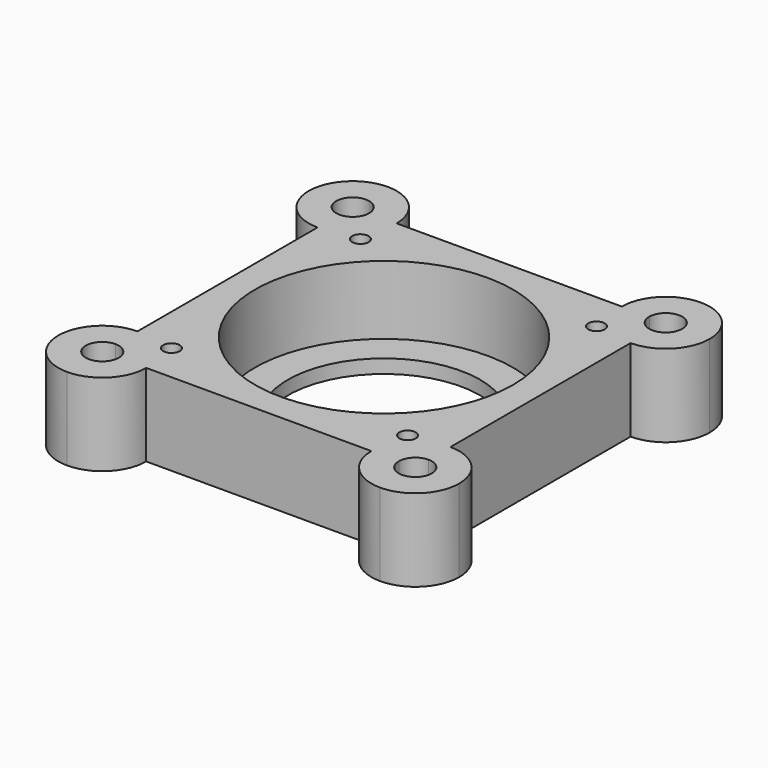
from build123d import *

# Parameters (mm, degrees)
F0_R     = 1.5
F0_R_2   = 23.5
F1_DEPTH = 15
F0_R_3   = 17.5
F2_DEPTH = 2.5
F3_SIZE  = 2


# Not quite as in the source:
# - a feature names something its author has since deleted; it is built from what else it names


with BuildPart() as f1:
    # F0 (on Top) → F1 (new body)
    with BuildSketch(Plane.XY):
        with BuildLine():
            Line((-28.5, 25.5), (-28.5, 20.5))
            ThreePointArc((-28.5, 20.5), (-22.8431457505, 22.8431457505), (-20.5, 28.5))
            Line((-20.5, 28.5), (-25.5, 28.5))
            ThreePointArc((-25.5, 28.5), (-26.3786796564, 26.3786796564), (-28.5, 25.5))
        make_face()
        with BuildLine():
            Line((-20.5, -28.5), (20.5, -28.5))
            ThreePointArc((20.5, -28.5), (22.8431457505, -22.8431457505), (28.5, -20.5))
            Line((28.5, -20.5), (28.5, 20.5))
            ThreePointArc((28.5, 20.5), (22.8431457505, 22.8431457505), (20.5, 28.5))
            Line((20.5, 28.5), (-20.5, 28.5))
            ThreePointArc((-20.5, 28.5), (-22.8431457505, 22.8431457505), (-28.5, 20.5))
            Line((-28.5, 20.5), (-28.5, -20.5))
            ThreePointArc((-28.5, -20.5), (-22.8431457505, -22.8431457505), (-20.5, -28.5))
        make_face()
        with Locations((-21.5, -21.5)):
            Circle(F0_R, mode=Mode.SUBTRACT)
        with Locations((21.5, -21.5)):
            Circle(F0_R, mode=Mode.SUBTRACT)
        with Locations((-21.5, 21.5)):
            Circle(F0_R, mode=Mode.SUBTRACT)
        Circle(F0_R_2, mode=Mode.SUBTRACT)
        with Locations((21.5, 21.5)):
            Circle(F0_R, mode=Mode.SUBTRACT)
        with BuildLine():
            ThreePointArc((20.5, 28.5), (22.8431457505, 22.8431457505), (28.5, 20.5))
            Line((28.5, 20.5), (28.5, 25.5))
            ThreePointArc((28.5, 25.5), (26.3786796564, 26.3786796564), (25.5, 28.5))
            Line((25.5, 28.5), (20.5, 28.5))
        make_face()
        with BuildLine():
            ThreePointArc((28.5, 20.5), (34.1568542495, 22.8431457505), (36.5, 28.5))
            ThreePointArc((36.5, 28.5), (34.1568542495, 34.1568542495), (28.5, 36.5))
            ThreePointArc((28.5, 36.5), (22.8431457505, 34.1568542495), (20.5, 28.5))
            Line((20.5, 28.5), (25.5, 28.5))
            ThreePointArc((25.5, 28.5), (28.5, 31.5), (31.5, 28.5))
            ThreePointArc((31.5, 28.5), (30.6213203436, 26.3786796564), (28.5, 25.5))
            Line((28.5, 25.5), (28.5, 20.5))
        make_face()
        with BuildLine():
            ThreePointArc((20.5, -28.5), (22.8431457505, -34.1568542495), (28.5, -36.5))
            ThreePointArc((28.5, -36.5), (34.1568542495, -34.1568542495), (36.5, -28.5))
            ThreePointArc((36.5, -28.5), (34.1568542495, -22.8431457505), (28.5, -20.5))
            Line((28.5, -20.5), (28.5, -25.5))
            ThreePointArc((28.5, -25.5), (30.6213203436, -26.3786796564), (31.5, -28.5))
            ThreePointArc((31.5, -28.5), (28.5, -31.5), (25.5, -28.5))
            Line((25.5, -28.5), (20.5, -28.5))
        make_face()
        with BuildLine():
            ThreePointArc((28.5, -20.5), (22.8431457505, -22.8431457505), (20.5, -28.5))
            Line((20.5, -28.5), (25.5, -28.5))
            ThreePointArc((25.5, -28.5), (26.3786796564, -26.3786796564), (28.5, -25.5))
            Line((28.5, -25.5), (28.5, -20.5))
        make_face()
        with BuildLine():
            Line((-25.5, -28.5), (-20.5, -28.5))
            ThreePointArc((-20.5, -28.5), (-22.8431457505, -22.8431457505), (-28.5, -20.5))
            Line((-28.5, -20.5), (-28.5, -25.5))
            ThreePointArc((-28.5, -25.5), (-26.3786796564, -26.3786796564), (-25.5, -28.5))
        make_face()
        with BuildLine():
            ThreePointArc((-36.5, -28.5), (-34.1568542495, -34.1568542495), (-28.5, -36.5))
            ThreePointArc((-28.5, -36.5), (-22.8431457505, -34.1568542495), (-20.5, -28.5))
            Line((-20.5, -28.5), (-25.5, -28.5))
            ThreePointArc((-25.5, -28.5), (-30.6213203436, -30.6213203436), (-28.5, -25.5))
            Line((-28.5, -25.5), (-28.5, -20.5))
            ThreePointArc((-28.5, -20.5), (-34.1568542495, -22.8431457505), (-36.5, -28.5))
        make_face()
        with BuildLine():
            ThreePointArc((-28.4999999613, 36.5), (-34.1568542358, 34.1568542632), (-36.5, 28.5))
            ThreePointArc((-36.5, 28.5), (-34.1568542495, 22.8431457505), (-28.5, 20.5))
            Line((-28.5, 20.5), (-28.5, 25.5))
            ThreePointArc((-28.5, 25.5), (-30.6213203436, 30.6213203436), (-25.5, 28.5))
            Line((-25.5, 28.5), (-20.5, 28.5))
            ThreePointArc((-20.5, 28.5), (-22.8431457368, 34.1568542358), (-28.4999999613, 36.5))
        make_face()
    extrude(amount=F1_DEPTH)

    # F0 (on Top) → F2 (join)
    with BuildSketch(Plane.XY):
        Circle(F0_R_2)
        Circle(F0_R_3, mode=Mode.SUBTRACT)
    extrude(amount=F2_DEPTH)

    # F3
    f3_edges = [f1.edges().sort_by_distance(p)[0] for p in [
        (31.5, 28.5, 0),
        (-28.5, 31.5, 0),
        (-31.5, -28.5, 0),
        (28.5, -31.5, 0),
    ]]
    chamfer(f3_edges, length=F3_SIZE)


solid = f1.part
